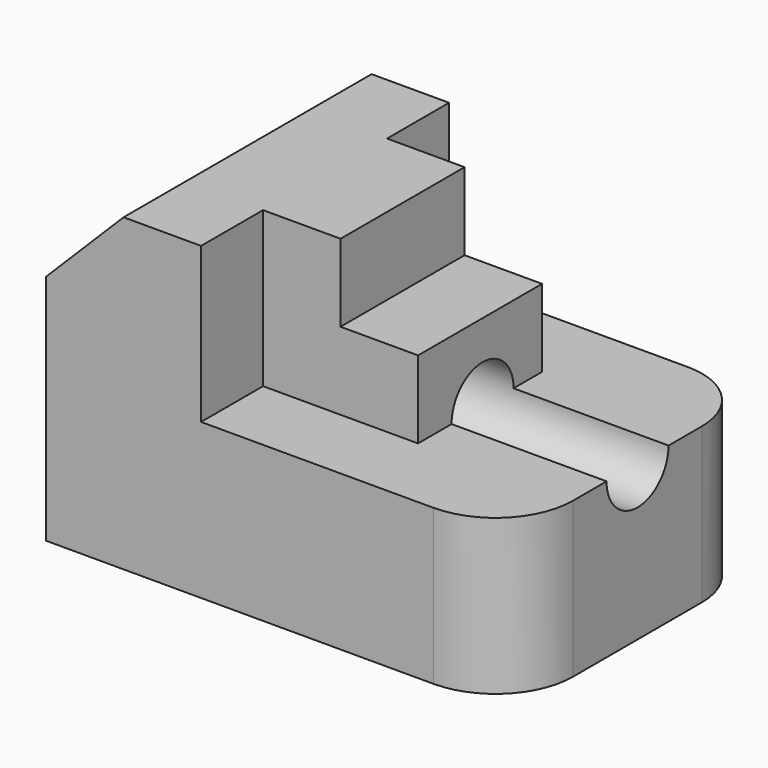
from build123d import *

# Parameters (mm, degrees)
F1_DEPTH  = 25.4
F3_DEPTH  = 50.801
F4_W      = 25.4
F4_H      = 12.7
F5_DEPTH  = 25.4
F6_W      = 25.4
F6_H      = 50.8
F7_DEPTH  = 25.4
F8_W      = 12.7
F8_H      = 25.4
F9_DEPTH  = 12.7
F10_DEPTH = 50.801
F12_DEPTH = 76.201


with BuildPart() as f1:
    # F0 (on Top) → F1 (new body, symmetric)
    with BuildSketch(Plane.XY):
        with BuildLine():
            Line((0, 50.8), (0, 0))
            Line((0, 0), (76.2, 0))
            Line((76.2, 0), (76.2, 39.1281142461))
            ThreePointArc((76.2, 39.1281142461), (72.7813838119, 47.3813838119), (64.5281142461, 50.8))
            Line((64.5281142461, 50.8), (0, 50.8))
        make_face()
    extrude(amount=F1_DEPTH, both=True)

    # F2 (on face) → F3 (cut, through all)
    with BuildSketch(Plane.XZ):
        Polygon((12.7, 25.4), (0, 25.4), (0, 12.7), align=None)
    extrude(amount=-F3_DEPTH, mode=Mode.SUBTRACT)

    # F4 (on face) → F5 (cut)
    with BuildSketch(Plane.XY.offset(25.4)):
        with Locations((38.1, 44.45)):
            Rectangle(F4_W, F4_H)
        with Locations((38.1, 6.35)):
            Rectangle(F4_W, F4_H)
    extrude(amount=-F5_DEPTH, mode=Mode.SUBTRACT)

    # F6 (on face) → F7 (cut, through all)
    with BuildSketch(Plane.XY.offset(25.4)):
        with Locations((63.5, 25.4)):
            Rectangle(F6_W, F6_H)
    extrude(amount=-F7_DEPTH, mode=Mode.SUBTRACT)

    # F8 (on face) → F9 (cut)
    with BuildSketch(Plane.XY.offset(25.4)):
        with Locations((44.45, 25.4)):
            Rectangle(F8_W, F8_H)
    extrude(amount=-F9_DEPTH, mode=Mode.SUBTRACT)

    # F4 (on face) → F10 (cut, through all)
    with BuildSketch(Plane.XY.offset(25.4)):
        with BuildLine():
            Line((76.2, 0), (76.2, 12.7))
            ThreePointArc((76.2, 12.7), (72.4802561211, 3.7197438789), (63.5, 0))
            Line((63.5, 0), (76.2, 0))
        make_face()
    extrude(amount=-F10_DEPTH, mode=Mode.SUBTRACT)

    # F11 (on face) → F12 (cut, through all)
    with BuildSketch(Plane.YZ.offset(76.2)):
        with BuildLine():
            Line((19.564057123, 0), (32.264057123, 0))
            ThreePointArc((32.264057123, 0), (25.914057123, 6.35), (19.564057123, 0))
        make_face()
        with BuildLine():
            ThreePointArc((19.564057123, 0), (25.914057123, -6.35), (32.264057123, 0))
            Line((32.264057123, 0), (19.564057123, 0))
        make_face()
    extrude(amount=-F12_DEPTH, mode=Mode.SUBTRACT)


solid = f1.part
